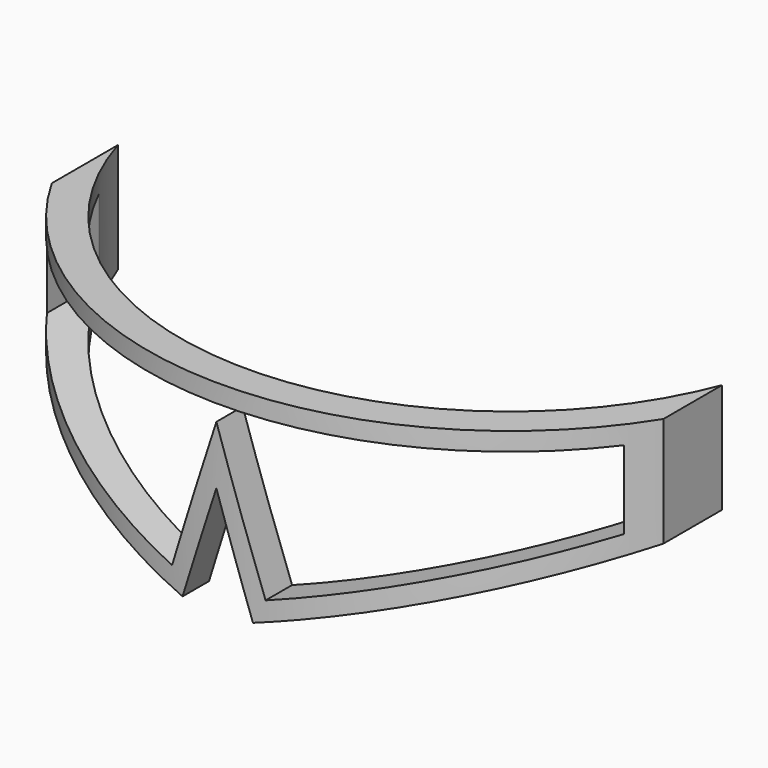
from build123d import *

# Parameters (mm, degrees)
F1_DEPTH = 75
F4_DEPTH = 200
F5_DEPTH = 100


# Not quite as in the source:
# - ends of sketch curves that miss each other by under 0.0002 mm in the source are joined


with BuildPart() as f1:
    # F0 (on Front) → F1 (new body, symmetric)
    with BuildSketch(Plane.XZ):
        Polygon((64.9607930725, 65.0385569036), (-20.0392069275, 65.0385569036), (-105.0392069275, 65.0385569036), (-105.0392069275, 35.0244045258), (-29.7518869333, 10.1945746155), (-20.0392069275, 39.6446734667), (-10.3405706844, 10.2371571158), (64.9607930725, 35.0385569036), align=None)
    extrude(amount=F1_DEPTH, both=True)

    # F2 (on face) → F4 (cut)
    with BuildSketch(Plane.XZ.offset(75)):
        Polygon((-100.0392069275, 38.640326764), (-32.9342746626, 16.5090348727), (-20.0392069275, 55.6085438923), (-7.1575624177, 16.5497358238), (59.9607930725, 38.6559645103), (59.9607930725, 60.0385569036), (-100.0392069275, 60.0385569036), align=None)
    extrude(amount=-F4_DEPTH, mode=Mode.SUBTRACT)

    # F3 (on face) → F5 (intersect)
    with BuildSketch(Plane.XY.offset(65.0385569036)):
        with BuildLine():
            Line((-107.177117556, 42.4698600353), (-115.9930899739, 40.6591594219))
            ThreePointArc((-115.9930899739, 40.6591594219), (-18.9798846841, -38.4537255363), (78.0333206058, 40.6591594219))
            Line((78.0333206058, 40.6591594219), (69.2173481878, 42.4698600353))
            ThreePointArc((69.2173481878, 42.4698600353), (-18.9798846841, -29.4537251816), (-107.177117556, 42.4698600353))
        make_face()
    extrude(amount=-F5_DEPTH, mode=Mode.INTERSECT)


solid = f1.part
